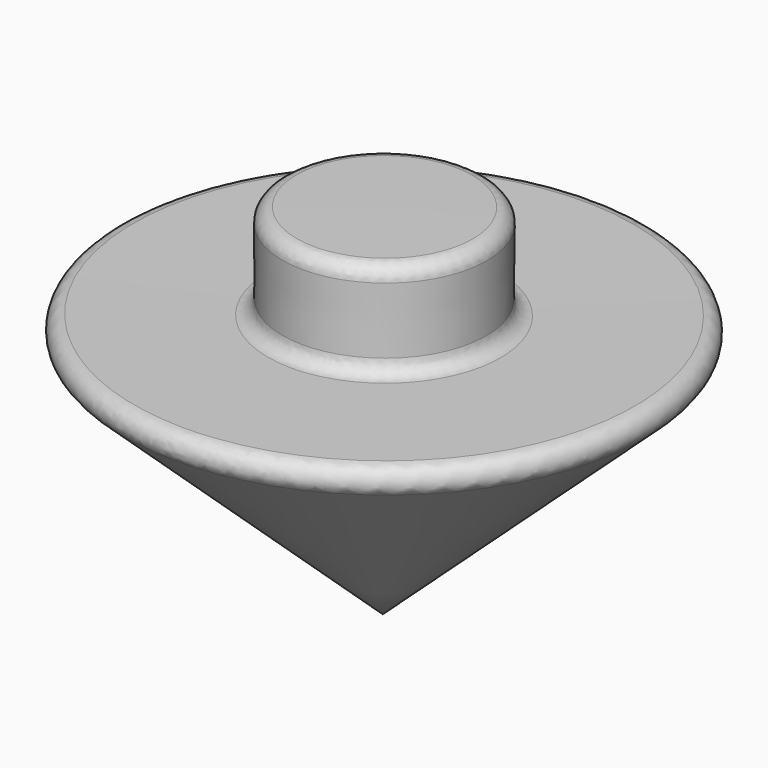
from build123d import *

# Parameters (mm, degrees)
F4_R = 1.27
F5_R = 1.27


# Not quite as in the source:
# - the program builds the solid bodies; features that only make, move or delete a surface that nothing else refers to are left out


with BuildPart() as f1:
    # F0 (on Right) → F1 (revolve)
    with BuildSketch(Plane.YZ):
        Polygon((-25.1451414078, 23.3748648316), (0, 0), (0.1911758445, 31.6073447466), (-8.8075501844, 31.6073447466), (-8.8075501844, 23.2158955187), align=None)
    revolve(axis=Axis((0, 0.0955879223, 15.8036723733), (0, -0.006048352, -0.9999817086)))

    # F4
    f4_edges = [f1.edges().sort_by_distance(p)[0] for p in [
        (0, 25.426055, 23.068987),
    ]]
    fillet(f4_edges, radius=F4_R)

    # F5
    f5_edges = [f1.edges().sort_by_distance(p)[0] for p in [
        (0, 9.189243, 31.498492),
        (0, 9.087736, 23.107657),
        (0, -8.80755, 27.41162),
        (0, -15.337301, 23.279432),
        (0, 22.14782, 23.076746),
    ]]
    fillet(f5_edges, radius=F5_R)


solid = f1.part
